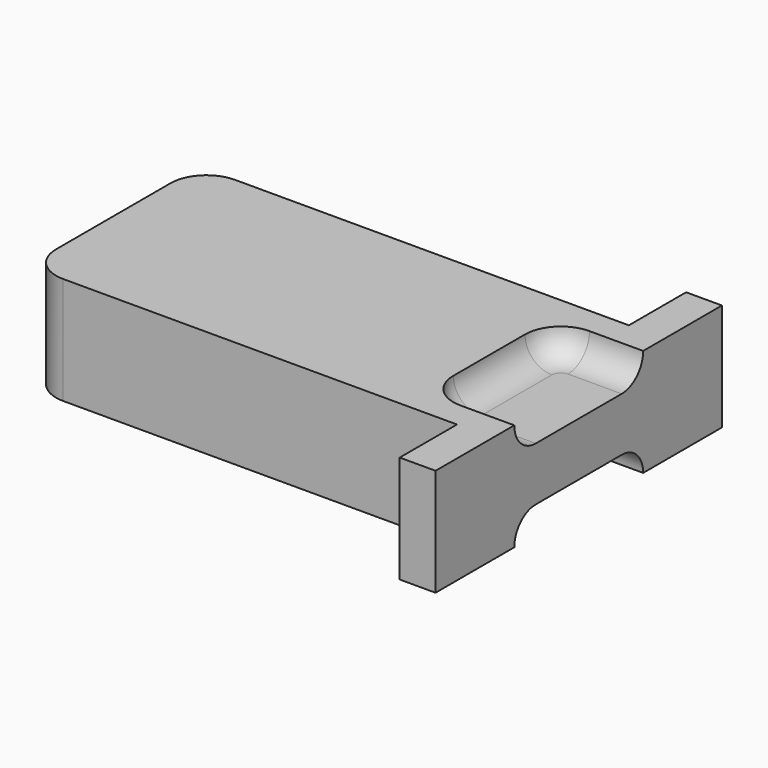
from build123d import *

# Parameters (mm, degrees)
F1_DEPTH = 9.525
F2_R     = 6.35
F4_DEPTH = 4.7625
F5_R     = 4.76249
F7_DEPTH = 4.7625
F8_R     = 4.76249


# Not quite as in the source:
# - a fillet or chamfer is up to 0.001 mm smaller than in the source, because OpenCascade refuses the exact size


with BuildPart() as f1:
    # F0 (on Top) → F1 (new body, symmetric)
    with BuildSketch(Plane.XY):
        Polygon((-82.55, 19.05), (-82.55, -19.05), (-6.35, -19.05), (-6.35, -31.75), (0, -31.75), (0, 31.75), (-6.35, 31.75), (-6.35, 19.05), align=None)
    extrude(amount=F1_DEPTH, both=True)

    # F2
    f2_edges = [f1.edges().sort_by_distance(p)[0] for p in [
        (-82.55, -19.05, 0),
        (-82.55, 19.05, 0),
    ]]
    fillet(f2_edges, radius=F2_R)

    # F3 (on face) → F4 (cut)
    with BuildSketch(Plane.XY.offset(9.525)):
        with BuildLine():
            Line((0, -14.2875), (0, 14.2875))
            Line((0, 14.2875), (-9.525, 14.2875))
            ThreePointArc((-9.525, 14.2875), (-14.0151280605, 12.4276280605), (-15.875, 7.9375))
            Line((-15.875, 7.9375), (-15.875, -7.9375))
            ThreePointArc((-15.875, -7.9375), (-14.0151280605, -12.4276280605), (-9.525, -14.2875))
            Line((-9.525, -14.2875), (0, -14.2875))
        make_face()
    extrude(amount=-F4_DEPTH, mode=Mode.SUBTRACT)

    # F5 (radius 4.7625 in the source; OpenCascade refuses exactly that, so slightly less here)
    f5_edges = [f1.edges().sort_by_distance(p)[0] for p in [
        (-4.7625, 14.2875, 4.7625),
        (-14.015128, 12.427628, 4.7625),
    ]]
    fillet(f5_edges, radius=F5_R)

    # F6 (on face) → F7 (cut)
    with BuildSketch(Plane(origin=(0, 0, -9.525), x_dir=(1, 0, 0), z_dir=(0, 0, -1))):
        with BuildLine():
            Line((0, -14.2875), (0, 14.2875))
            Line((0, 14.2875), (-9.525, 14.2875))
            ThreePointArc((-9.525, 14.2875), (-14.0151280605, 12.4276280605), (-15.875, 7.9375))
            Line((-15.875, 7.9375), (-15.875, -7.9375))
            ThreePointArc((-15.875, -7.9375), (-14.0151280605, -12.4276280605), (-9.525, -14.2875))
            Line((-9.525, -14.2875), (0, -14.2875))
        make_face()
    extrude(amount=-F7_DEPTH, mode=Mode.SUBTRACT)

    # F8 (radius 4.7625 in the source; OpenCascade refuses exactly that, so slightly less here)
    f8_edges = [f1.edges().sort_by_distance(p)[0] for p in [
        (-4.7625, -14.2875, -4.7625),
        (-14.015128, -12.427628, -4.7625),
    ]]
    fillet(f8_edges, radius=F8_R)


solid = f1.part
